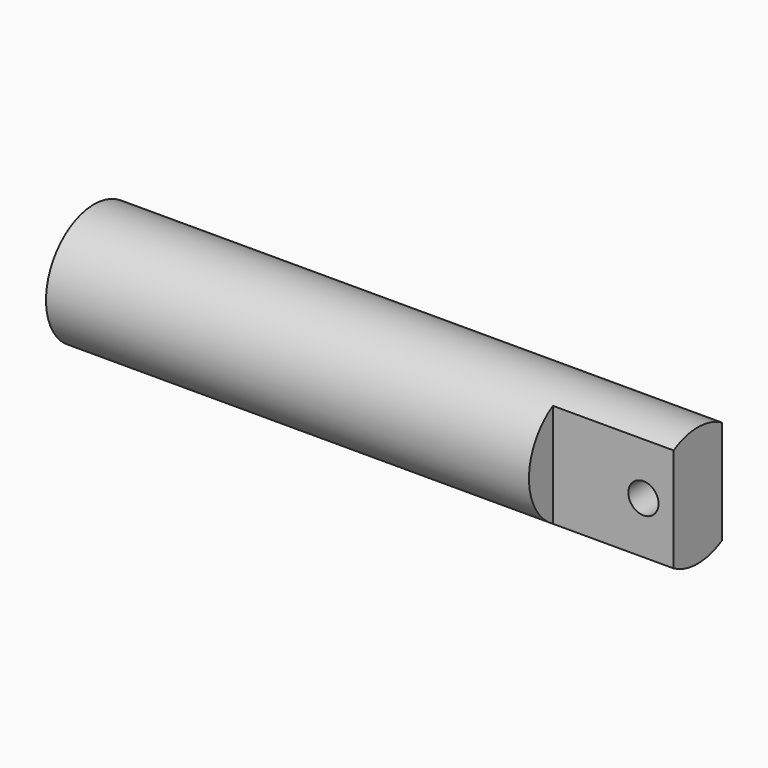
from build123d import *
from build123d import SkipClean  # not in build123d's __all__

# Parameters (mm, degrees)
F0_R     = 4.975
F1_DEPTH = 50
F3_DEPTH = 10
F4_R     = 1.25
F5_DEPTH = 5


with BuildPart() as f1:
    # F0 (on Right) → F1 (new body)
    with BuildSketch(Plane.YZ):
        Circle(F0_R)
    extrude(amount=F1_DEPTH)

    # F2 (on face) → F3 (cut)
    with BuildSketch(Plane.YZ.offset(50)):
        with BuildLine():
            Line((2.5, 4.3012352877), (2.5, -4.3012352877))
            ThreePointArc((2.5, -4.3012352877), (4.3120833132, -2.4812421285), (4.975, 0))
            ThreePointArc((4.975, 0), (4.3120833132, 2.4812421285), (2.5, 4.3012352877))
        make_face()
        with BuildLine():
            ThreePointArc((-2.5, 4.3012352877), (-4.975, 0), (-2.5, -4.3012352877))
            Line((-2.5, -4.3012352877), (-2.5, 4.3012352877))
        make_face()
    extrude(amount=-F3_DEPTH, mode=Mode.SUBTRACT)

    # F4 (on face) → F5 (cut)
    with BuildSketch(Plane(origin=(0, 2.5, 0), x_dir=(-1, 0, 0), z_dir=(0, 1, 0))):
        with Locations((-47.5, 0)):
            Circle(F4_R)
    extrude(amount=-F5_DEPTH, mode=Mode.SUBTRACT)

    # F6 (on Front) → F7 (revolve, cut)
    with BuildSketch(Plane.XZ):
        with BuildLine():
            Line((-2.5, 5), (-2.5, -5))
            ThreePointArc((-2.5, -5), (2.5, 0), (-2.5, 5))
        make_face()
    with SkipClean():  # cleaning this boolean's faces spoils the solid; the shape is the same uncleaned
        revolve(axis=Axis((-2.5, 0, 0), (0, 0, 1)), mode=Mode.SUBTRACT)


solid = f1.part
